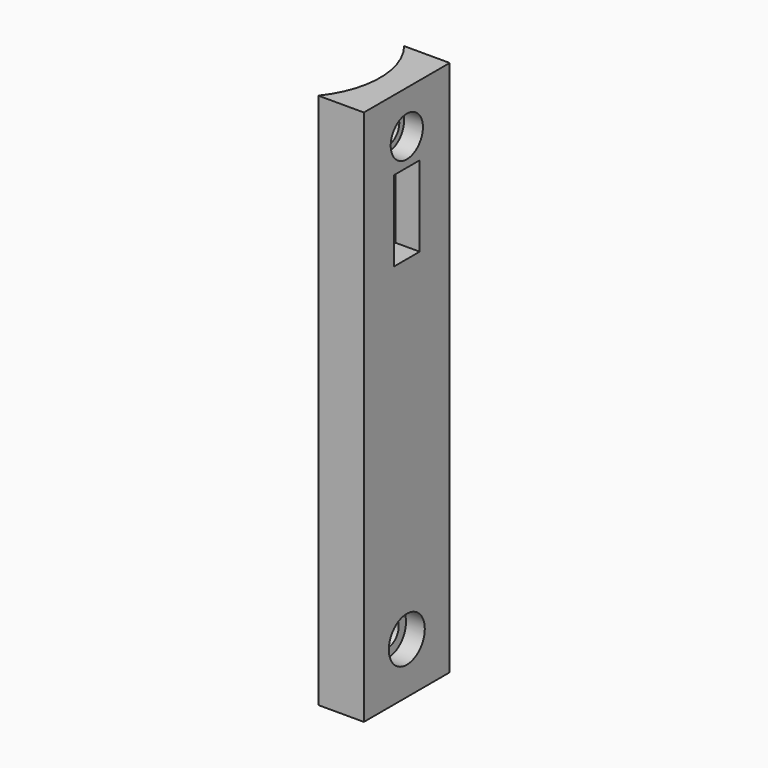
from build123d import *
from build123d import SkipClean  # not in build123d's __all__

# Parameters (mm, degrees)
F0_W      = 40
F0_H      = 200
F1_DEPTH  = 17
F2_R      = 32
F3_DEPTH  = 187
F4_DEPTH  = 195
F5_R      = 8.3828490824
F5_R_2    = 7.5
F6_DEPTH  = 7
F7_R      = 5
F7_R_2    = 5.25
F8_DEPTH  = 25
F9_W      = 12
F9_H      = 30
F10_DEPTH = 9


with BuildPart() as f1:
    # F0 (on Right) → F1 (new body)
    with BuildSketch(Plane.YZ):
        with Locations((19.5646310411, 53.8327481339)):
            Rectangle(F0_W, F0_H)
    extrude(amount=F1_DEPTH)

    # F2 (on Top) → F3 (cut, symmetric)
    with BuildSketch(Plane.XY):
        with Locations((-24.9799919936, 19.5646310411)):
            Circle(F2_R)
    extrude(amount=F3_DEPTH, both=True, mode=Mode.SUBTRACT)

    # F2 (on Top) → F4 (cut)
    with BuildSketch(Plane.XY):
        with Locations((-24.9799919936, 19.5646310411)):
            Circle(F2_R)
    extrude(amount=-F4_DEPTH, mode=Mode.SUBTRACT)

    # F5 (on face) → F6 (cut)
    with BuildSketch(Plane.YZ.offset(17)):
        with Locations((19.5646310411, -27.1672518661)):
            Circle(F5_R)
        with Locations((19.5646310411, 137.8327481339)):
            Circle(F5_R_2)
    extrude(amount=-F6_DEPTH, mode=Mode.SUBTRACT)

    # F7 (on face) → F8 (cut)
    with BuildSketch(Plane.YZ.offset(10)):
        with Locations((19.5646310411, -27.1672518661)):
            Circle(F7_R)
        with Locations((19.5646310411, 137.8327481339)):
            Circle(F7_R_2)
    with SkipClean():  # cleaning this boolean's faces spoils the solid; the shape is the same uncleaned
        extrude(amount=-F8_DEPTH, mode=Mode.SUBTRACT)

    # F9 (on face) → F10 (cut)
    with BuildSketch(Plane.YZ.offset(17)):
        with Locations((19.5646310411, 112.5827481339)):
            Rectangle(F9_W, F9_H)
    with SkipClean():  # cleaning this boolean's faces spoils the solid; the shape is the same uncleaned
        extrude(amount=-F10_DEPTH, mode=Mode.SUBTRACT)


solid = f1.part
